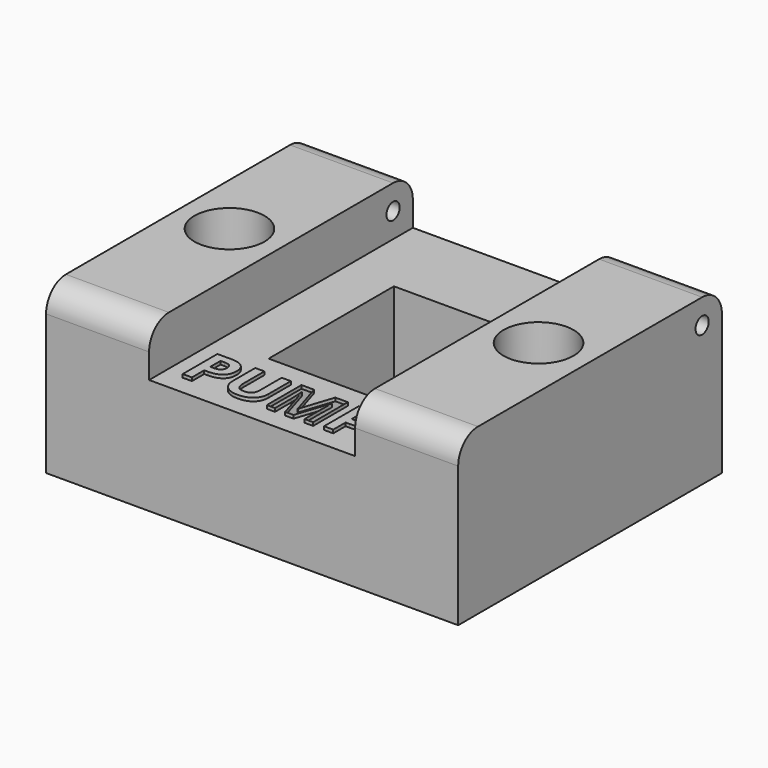
from build123d import *

# Parameters (mm, degrees)
F0_W          = 50
F0_H          = 40
F1_DEPTH      = 14
F2_W          = 12.8
F2_H          = 19
F3_DEPTH      = 14
F4_W          = 12.5
F4_H          = 40
F5_DEPTH      = 6
F6_R          = 2.1
F7_DEPTH      = 20
F8_R          = 4.25
F8_R_2        = 2.1
F9_DEPTH      = 6
F10_R         = 4.25
F11_DEPTH     = 6
F12_R         = 1
F13_DEPTH     = 50.001
F14_R         = 3
F15_TEXT_SIZE = 7.3702837754
F16_DEPTH     = 0.4


# Not quite as in the source:
# - Text() gives the source's letters only with a copy of the font that has no kerning and outlines rounded to 1/6400 em; it was checked with that copy


with BuildPart() as f1:
    # F0 (on Top) → F1 (new body)
    with BuildSketch(Plane.XY):
        Rectangle(F0_W, F0_H)
    extrude(amount=F1_DEPTH)

    # F2 (on face) → F3 (cut, through all)
    with BuildSketch(Plane.XY.offset(14)):
        Rectangle(F2_W, F2_H)
    extrude(amount=-F3_DEPTH, mode=Mode.SUBTRACT)

    # F4 (on face) → F5 (join)
    with BuildSketch(Plane.XY.offset(14)):
        with Locations((-18.75, 0)):
            Rectangle(F4_W, F4_H)
        with Locations((18.75, 0)):
            Rectangle(F4_W, F4_H)
    extrude(amount=F5_DEPTH)

    # F6 (on face) → F7 (cut, through all)
    with BuildSketch(Plane.XY.offset(20)):
        with Locations((-18.75, 0)):
            Circle(F6_R)
        with Locations((18.75, 0)):
            Circle(F6_R)
    extrude(amount=-F7_DEPTH, mode=Mode.SUBTRACT)

    # F8 (on face) → F9 (cut)
    with BuildSketch(Plane.XY.offset(20)):
        with Locations((-18.75, 0)):
            Circle(F8_R)
        with Locations((-18.75, 0)):
            Circle(F8_R_2, mode=Mode.SUBTRACT)
    extrude(amount=-F9_DEPTH, mode=Mode.SUBTRACT)

    # F10 (on face) → F11 (cut)
    with BuildSketch(Plane.XY.offset(20)):
        with Locations((18.75, 0)):
            Circle(F10_R)
    extrude(amount=-F11_DEPTH, mode=Mode.SUBTRACT)

    # F12 (on face) → F13 (cut, through all)
    with BuildSketch(Plane.YZ.offset(25)):
        with Locations((17, 17)):
            Circle(F12_R)
    extrude(amount=-F13_DEPTH, mode=Mode.SUBTRACT)

    # F14
    f14_edges = [f1.edges().sort_by_distance(p)[0] for p in [
        (18.75, 20, 20),
        (-18.75, 20, 20),
        (-18.75, -20, 20),
        (18.75, -20, 20),
    ]]
    fillet(f14_edges, radius=F14_R)

    # F15 (on face) → F16 (join)
    with BuildSketch(Plane.XY.offset(14)):
        with Locations((-10.965352878, -17.6489865407)):
            Text('PUMP', F15_TEXT_SIZE, font='Open Sans', font_style=FontStyle.BOLD, text_align=(TextAlign.LEFT, TextAlign.BOTTOM))
    extrude(amount=F16_DEPTH)


solid = f1.part
